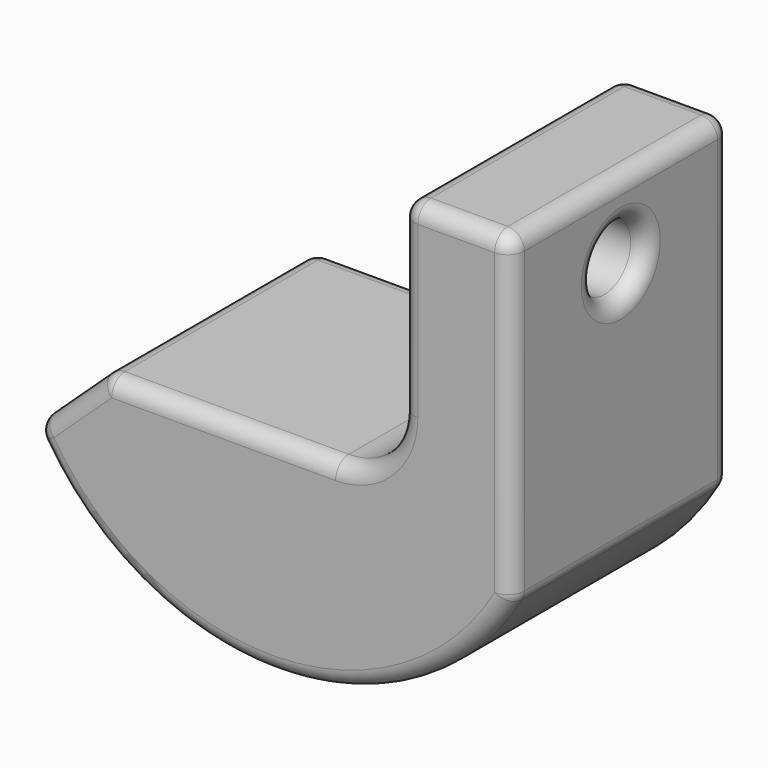
from build123d import *

# Parameters (mm, degrees)
F1_DEPTH = 6.35
F3_D     = 1.524
F4_R     = 0.381


with BuildPart() as f1:
    # F0 (on Front) → F1 (new body)
    with BuildSketch(Plane.XZ):
        with BuildLine():
            Line((0, -7.4092204591), (0, 0))
            Line((0, 0), (-2.54, 0))
            Line((-2.54, 0), (-2.54, -4.318))
            ThreePointArc((-2.54, -4.318), (-2.9863692655, -5.3956307345), (-4.064, -5.842))
            Line((-4.064, -5.842), (-9.398, -5.842))
            Line((-9.398, -5.842), (-11.068511021, -7.3997767286))
            ThreePointArc((-11.068511021, -7.3997767286), (-5.53701683, -10.6408992323), (0, -7.4092204591))
        make_face()
    extrude(amount=F1_DEPTH)

    # F3 (through all)
    with Locations(Plane.YZ):
        with Locations((-3.175, -1.7639952663)):
            Hole(F3_D / 2)

    # F4
    f4_edges = [f1.edges().sort_by_distance(p)[0] for p in [
        (-2.54, -3.175, 0),
        (0, -3.175, 0),
        (-1.27, -6.35, 0),
        (-1.27, 0, 0),
        (0, -6.35, -3.70461),
        (-2.54, -6.35, -2.159),
        (-2.986369, -6.35, -5.395631),
        (-6.731, -6.35, -5.842),
        (-10.233256, -6.35, -6.620888),
        (-5.537017, -6.35, -10.640899),
        (0, -3.175, -7.40922),
        (-9.398, -3.175, -5.842),
        (-2.54, 0, -2.159),
        (-2.986369, 0, -5.395631),
        (-6.731, 0, -5.842),
        (-10.233256, 0, -6.620888),
        (-5.537017, 0, -10.640899),
        (0, 0, -3.70461),
        (-11.068511, -3.175, -7.399777),
        (0, -3.937, -1.763995),
        (-2.54, -3.937, -1.763995),
    ]]
    fillet(f4_edges, radius=F4_R)


solid = f1.part
